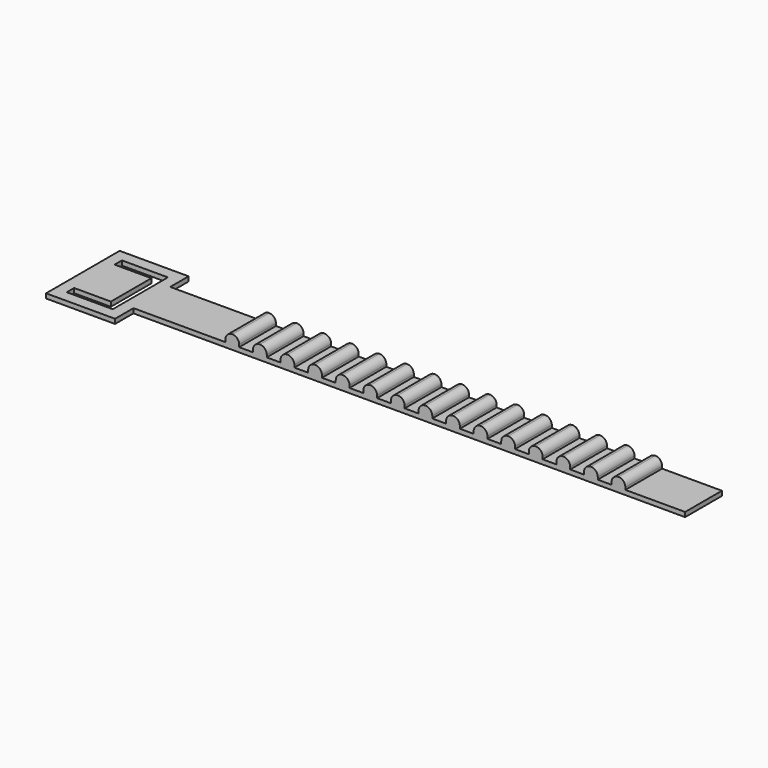
from build123d import *

# Parameters (mm, degrees)
F0_W     = 120
F0_H     = 10
F1_DEPTH = 1
F2_W     = 3
F2_H     = 10
F3_DEPTH = 3
F4_R     = 1.5
F5_R     = 1.49999
F6_R     = 1.49999


# Not quite as in the source:
# - a fillet or chamfer is up to 0.001 mm smaller than in the source, because OpenCascade refuses the exact size


with BuildPart() as f1:
    # F0 (on Top) → F1 (new body)
    with BuildSketch(Plane.XY):
        Rectangle(F0_W, F0_H)
        Polygon((-60, -5), (-60, 5), (-60, 10), (-75, 10), (-75, -10), (-60, -10), align=None)
        Polygon((-72.5, 5.5), (-72.5, 7.5), (-62.5, 7.5), (-62.5, -7.5), (-72.5, -7.5), (-72.5, -5.5), (-64.5, -5.5), (-64.5, 5.5), align=None, mode=Mode.SUBTRACT)
    extrude(amount=F1_DEPTH)

    # F2 (on Top) → F3 (join)
    with BuildSketch(Plane.XY):
        with Locations((-38.5, 0)):
            Rectangle(F2_W, F2_H)
        with Locations((-32.5, 0)):
            Rectangle(F2_W, F2_H)
        with Locations((-26.5, 0)):
            Rectangle(F2_W, F2_H)
        with Locations((-20.5, 0)):
            Rectangle(F2_W, F2_H)
        with Locations((-14.5, 0)):
            Rectangle(F2_W, F2_H)
        with Locations((-8.5, 0)):
            Rectangle(F2_W, F2_H)
        with Locations((-2.5, 0)):
            Rectangle(F2_W, F2_H)
        with Locations((3.5, 0)):
            Rectangle(F2_W, F2_H)
        with Locations((9.5, 0)):
            Rectangle(F2_W, F2_H)
        with Locations((15.5, 0)):
            Rectangle(F2_W, F2_H)
        with Locations((21.5, 0)):
            Rectangle(F2_W, F2_H)
        with Locations((27.5, 0)):
            Rectangle(F2_W, F2_H)
        with Locations((33.5, 0)):
            Rectangle(F2_W, F2_H)
        with Locations((39.5, 0)):
            Rectangle(F2_W, F2_H)
        with Locations((45.5, 0)):
            Rectangle(F2_W, F2_H)
    extrude(amount=F3_DEPTH)

    # F4
    f4_edges = [f1.edges().sort_by_distance(p)[0] for p in [
        (-40, 0, 3),
    ]]
    fillet(f4_edges, radius=F4_R)

    # F5 (radius 1.5 in the source; OpenCascade refuses exactly that, so slightly less here)
    f5_edges = [f1.edges().sort_by_distance(p)[0] for p in [
        (-37, 0, 3),
    ]]
    fillet(f5_edges, radius=F5_R)

    # F6 (radius 1.5 in the source; OpenCascade refuses exactly that, so slightly less here)
    f6_edges = [f1.edges().sort_by_distance(p)[0] for p in [
        (-34, 0, 3),
        (-31, 0, 3),
        (-28, 0, 3),
        (-25, 0, 3),
        (-22, 0, 3),
        (-19, 0, 3),
        (-16, 0, 3),
        (-13, 0, 3),
        (-10, 0, 3),
        (-7, 0, 3),
        (-4, 0, 3),
        (-1, 0, 3),
        (2, 0, 3),
        (5, 0, 3),
        (8, 0, 3),
        (11, 0, 3),
        (14, 0, 3),
        (17, 0, 3),
        (20, 0, 3),
        (23, 0, 3),
        (26, 0, 3),
        (29, 0, 3),
        (32, 0, 3),
        (35, 0, 3),
        (38, 0, 3),
        (41, 0, 3),
        (44, 0, 3),
        (47, 0, 3),
    ]]
    fillet(f6_edges, radius=F6_R)


solid = f1.part
